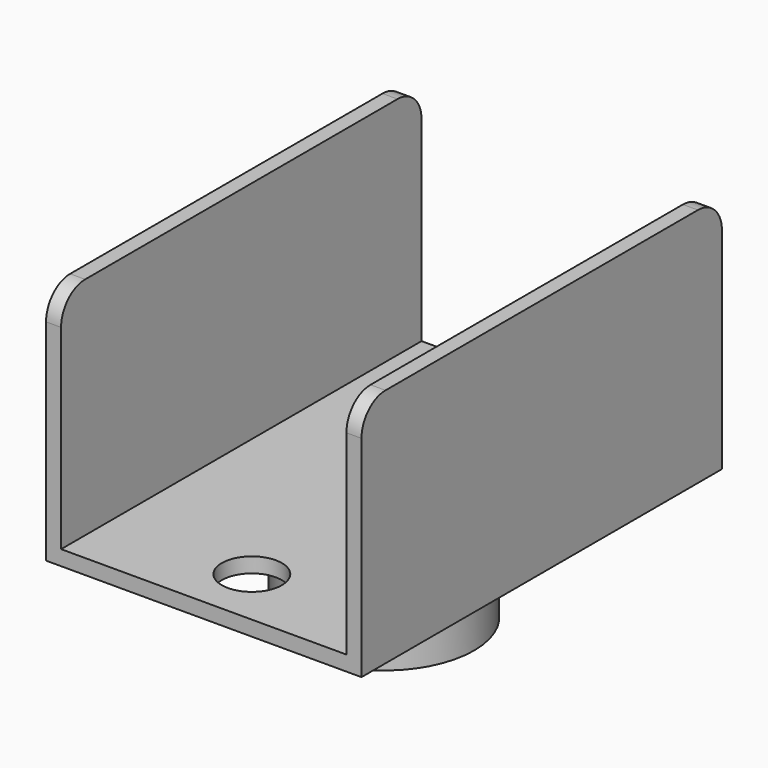
from build123d import *

# Parameters (mm, degrees)
F1_DEPTH = 30
F2_R     = 2.5
F3_DEPTH = 3
F4_R     = 6
F4_R_2   = 2.5
F5_DEPTH = 4
F6_R     = 2
F7_D     = 4
F7_DEPTH = 15
F7_TIP   = 1.2017212381


with BuildPart() as f1:
    # F0 (on Front) → F1 (new body)
    with BuildSketch(Plane.XZ):
        Polygon((0, 1), (0, 0), (21, 0), (21, 1), (21, 16), (20, 16), (20, 1), (1, 1), (1, 16), (0, 16), align=None)
    extrude(amount=-F1_DEPTH)

    # F2 (on face) → F3 (join)
    with BuildSketch(Plane.XY.offset(1)):
        with Locations((10.5, 15)):
            Circle(F2_R)
    extrude(amount=-F3_DEPTH)

    # F4 (on face) → F5 (join)
    with BuildSketch(Plane(origin=(0, 0, -2), x_dir=(1, 0, 0), z_dir=(0, 0, -1))):
        with Locations((10.5, -15)):
            Circle(F4_R)
        with Locations((10.5, -15)):
            Circle(F4_R_2, mode=Mode.SUBTRACT)
        with Locations((10.5, -15)):
            Circle(F4_R_2)
    extrude(amount=F5_DEPTH)

    # F6
    f6_edges = [f1.edges().sort_by_distance(p)[0] for p in [
        (20.5, 0, 16),
        (20.5, 30, 16),
        (0.5, 30, 16),
        (0.5, 0, 16),
    ]]
    fillet(f6_edges, radius=F6_R)

    # F7
    with Locations(Plane.XY.offset(1)):
        with Locations((10.5, 4), (10.5, 26)):
            Hole(F7_D / 2, depth=F7_DEPTH)
            with Locations((0, 0, -(F7_DEPTH + F7_TIP / 2))):  # 118° drill point
                Cone(0, F7_D / 2, F7_TIP, mode=Mode.SUBTRACT)


solid = f1.part
